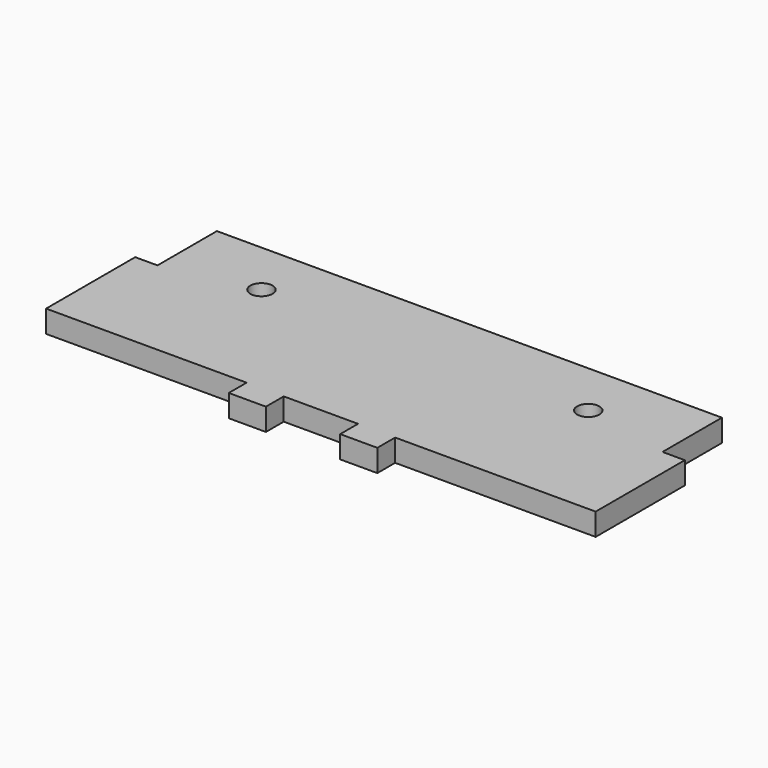
from build123d import *

# Parameters (mm, degrees)
F0_W     = 68
F0_H     = 25
F1_DEPTH = 3
F2_W     = 5
F2_H     = 3
F3_DEPTH = 3
F4_W     = 15
F4_H     = 3
F5_DEPTH = 3
F7_R     = 1.5
F8_DEPTH = 3


# Not quite as in the source:
# - a feature names something its author has since deleted; it is built from what else it names


with BuildPart() as f1:
    # F0 (on Top) → F1 (new body)
    with BuildSketch(Plane.XY):
        Rectangle(F0_W, F0_H)
    extrude(amount=F1_DEPTH)

    # F2 (on face) → F3 (join)
    with BuildSketch(Plane.XZ.offset(12.5)):
        with Locations((7.5, 1.5)):
            Rectangle(F2_W, F2_H)
    extrude(amount=F3_DEPTH)

    # F4 (on face) → F5 (join)
    with BuildSketch(Plane.YZ.offset(34)):
        with Locations((-5, 1.5)):
            Rectangle(F4_W, F4_H)
    extrude(amount=F5_DEPTH)

    # F6: F1 across plane


with BuildPart() as f1_1:
    add(f1.part)
    add(f1.part.mirror(Plane.YZ))

    # F7 (on face) → F8 (cut)
    with BuildSketch(Plane.XY.offset(3)):
        with Locations((22, 5)):
            Circle(F7_R)
        with Locations((-22, 5)):
            Circle(F7_R)
    extrude(amount=-F8_DEPTH, mode=Mode.SUBTRACT)


solid = f1_1.part
